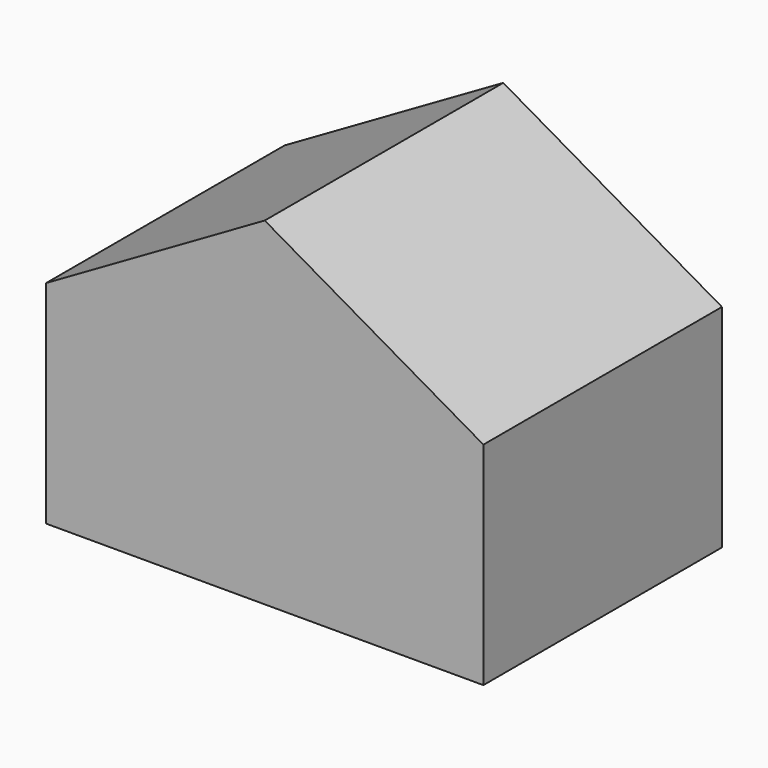
from build123d import *

# Parameters (mm, degrees)
F2_DEPTH = 381


# Not quite as in the source:
# - the program builds the solid bodies; features that only make, move or delete a surface that nothing else refers to are left out


with BuildPart() as f2:
    # F0 (on Front) → F2 (new body)
    with BuildSketch(Plane.XZ):
        Polygon((-279.4, 54.6750131028), (-279.4, -215.9), (279.4, -215.9), (279.4, 54.6750131028), (0, 215.9), align=None)
    extrude(amount=F2_DEPTH)


solid = f2.part
